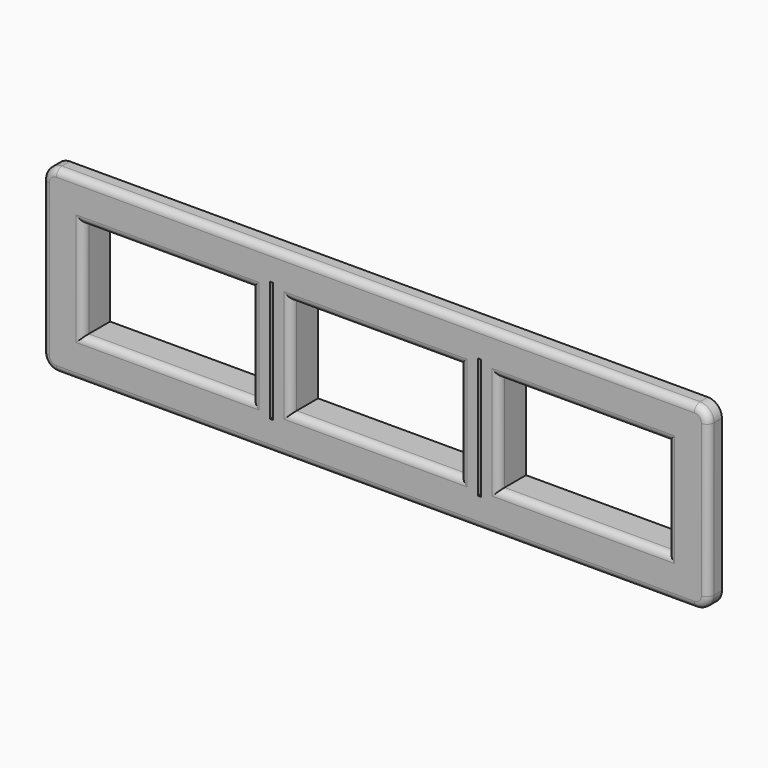
from build123d import *

# Parameters (mm, degrees)
F0_W          = 44.2
F0_H          = 9.6
F0_W_2        = 12
F0_H_2        = 7
F0_W_3        = 0.2
F0_H_3        = 8.6
F1_DEPTH      = 2.4
F2_R          = 0.5
F3_W          = 44.2
F3_H          = 1.2
F4_DEPTH      = 1.6
F5_W          = 44.2
F5_H          = 1.2
F6_DEPTH      = 1.6
F8_DEPTH      = 1.6
F10_DEPTH     = 1.6
F11_R         = 0.5
F12_T1_DEPTH  = 3.7
F12_T3_DEPTH  = 3.7
F12_T6_ANGLE  = 90
F12_T8_ANGLE  = 90
F12_T10_ANGLE = 90
F12_T12_ANGLE = 90


# Not quite as in the source:
# - a fillet or chamfer that OpenCascade refuses, or shapes differently, is made with other operations: its cross-section is extruded or revolved along the edge and cut away or added
# - a feature names something its author has since deleted; it is built from what else it names


with BuildPart() as f1:
    # F0 (on Front) → F1 (new body)
    with BuildSketch(Plane.XZ):
        with Locations((58.0827572465, 2.8)):
            Rectangle(F0_W, F0_H)
        with Locations((43.2827572465, 2.8)):
            Rectangle(F0_W_2, F0_H_2, mode=Mode.SUBTRACT)
        with Locations((50.6827572465, 2.8)):
            Rectangle(F0_W_3, F0_H_3, mode=Mode.SUBTRACT)
        with Locations((58.0827572465, 2.8)):
            Rectangle(F0_W_2, F0_H_2, mode=Mode.SUBTRACT)
        with Locations((65.4827572465, 2.8)):
            Rectangle(F0_W_3, F0_H_3, mode=Mode.SUBTRACT)
        with Locations((72.8827572465, 2.8)):
            Rectangle(F0_W_2, F0_H_2, mode=Mode.SUBTRACT)
    extrude(amount=F1_DEPTH)

    # F2
    f2_edges = [f1.edges().sort_by_distance(p)[0] for p in [
        (43.282757, -2.4, 6.3),
        (37.282757, -2.4, 2.8),
        (49.282757, -2.4, 2.8),
        (58.082757, -2.4, 6.3),
        (52.082757, -2.4, 2.8),
        (58.082757, -2.4, -0.7),
        (43.282757, -2.4, -0.7),
        (64.082757, -2.4, 2.8),
        (66.882757, -2.4, 2.8),
        (72.882757, -2.4, -0.7),
        (72.882757, -2.4, 6.3),
        (78.882757, -2.4, 2.8),
    ]]
    fillet(f2_edges, radius=F2_R)

    # F3 (on face) → F4 (join)
    with BuildSketch(Plane(origin=(0, 0, -2), x_dir=(1, 0, 0), z_dir=(0, 0, -1))):
        with Locations((58.0827572465, 1.8)):
            Rectangle(F3_W, F3_H)
    extrude(amount=F4_DEPTH)

    # F5 (on face) → F6 (join)
    with BuildSketch(Plane.XY.offset(7.6)):
        with Locations((58.0827572465, -1.8)):
            Rectangle(F5_W, F5_H)
    extrude(amount=F6_DEPTH)

    # F7 (on face) → F8 (join)
    with BuildSketch(Plane(origin=(35.9827572465, 0, 0), x_dir=(0, -1, 0), z_dir=(-1, 0, 0))):
        Polygon((2.4, -3.6), (2.4, 9.2), (1.2, 9.2), (1.2, 7.6), (1.2, -2), (1.2, -3.6), align=None)
    extrude(amount=F8_DEPTH)

    # F9 (on face) → F10 (join)
    with BuildSketch(Plane.YZ.offset(80.1827572465)):
        Polygon((-1.2, 9.2), (-2.4, 9.2), (-2.4, -3.6), (-1.2, -3.6), (-1.2, -2), (-1.2, 7.6), align=None)
    extrude(amount=F10_DEPTH)

    # F11
    f11_edges = [f1.edges().sort_by_distance(p)[0] for p in [
        (58.082757, -2.4, 9.2),
        (81.782757, -2.4, 2.8),
        (58.082757, -2.4, -3.6),
        (34.382757, -2.4, 2.8),
    ]]
    fillet(f11_edges, radius=F11_R)

    # F12: fillet of radius 1 on 8 edges, made by hand

    # F12_s2 → F12_t1 (cut)
    with BuildSketch(Plane.XZ.offset(-2.5)):
        with BuildLine():
            ThreePointArc((36.9827572465, 7.6), (36.2756504653, 7.3071067812), (35.9827572465, 6.6))
            Line((35.9827572465, 6.6), (35.9827572465, 7.6))
            Line((35.9827572465, 7.6), (36.9827572465, 7.6))
        make_face()
        with BuildLine():
            ThreePointArc((35.9827572465, -1), (36.2756504653, -1.7071067812), (36.9827572465, -2))
            Line((36.9827572465, -2), (35.9827572465, -2))
            Line((35.9827572465, -2), (35.9827572465, -1))
        make_face()
        with BuildLine():
            ThreePointArc((80.1827572465, -1), (79.8898640277, -1.7071067812), (79.1827572465, -2))
            Line((79.1827572465, -2), (80.1827572465, -2))
            Line((80.1827572465, -2), (80.1827572465, -1))
        make_face()
        with BuildLine():
            ThreePointArc((80.1827572465, 6.6), (79.8898640277, 7.3071067812), (79.1827572465, 7.6))
            Line((79.1827572465, 7.6), (80.1827572465, 7.6))
            Line((80.1827572465, 7.6), (80.1827572465, 6.6))
        make_face()
    extrude(amount=F12_T1_DEPTH, mode=Mode.SUBTRACT)

    # F12_s4 → F12_t3 (cut)
    with BuildSketch(Plane.XZ.offset(-1.3)):
        with BuildLine():
            ThreePointArc((80.7827572465, 9.2), (81.4898640277, 8.9071067812), (81.7827572465, 8.2))
            Line((81.7827572465, 8.2), (81.7827572465, 9.2))
            Line((81.7827572465, 9.2), (80.7827572465, 9.2))
        make_face()
        with BuildLine():
            ThreePointArc((81.7827572465, -2.6), (81.4898640277, -3.3071067812), (80.7827572465, -3.6))
            Line((80.7827572465, -3.6), (81.7827572465, -3.6))
            Line((81.7827572465, -3.6), (81.7827572465, -2.6))
        make_face()
        with BuildLine():
            ThreePointArc((34.3827572465, -2.6), (34.6756504653, -3.3071067812), (35.3827572465, -3.6))
            Line((35.3827572465, -3.6), (34.3827572465, -3.6))
            Line((34.3827572465, -3.6), (34.3827572465, -2.6))
        make_face()
        with BuildLine():
            ThreePointArc((35.3827572465, 9.2), (34.6756504653, 8.9071067812), (34.3827572465, 8.2))
            Line((34.3827572465, 8.2), (34.3827572465, 9.2))
            Line((34.3827572465, 9.2), (35.3827572465, 9.2))
        make_face()
    extrude(amount=F12_T3_DEPTH, mode=Mode.SUBTRACT)

    # F12_s5 → F12_t6 (revolve, cut)
    with BuildSketch(Plane.YZ.offset(35.3827572465)):
        with BuildLine():
            ThreePointArc((-2.4, 8.7), (-2.2535533906, 9.0535533906), (-1.9, 9.2))
            Line((-1.9, 9.2), (-2.4, 9.2))
            Line((-2.4, 9.2), (-2.4, 8.7))
        make_face()
    revolve(axis=Axis((35.3827572465, -2.4, 8.2), (0, -1, 0)), revolution_arc=F12_T6_ANGLE, mode=Mode.SUBTRACT)

    # F12_s7 → F12_t8 (revolve, cut)
    with BuildSketch(Plane.XY.offset(-2.6)):
        with BuildLine():
            ThreePointArc((34.8827572465, -2.4), (34.5292038559, -2.2535533906), (34.3827572465, -1.9))
            Line((34.3827572465, -1.9), (34.3827572465, -2.4))
            Line((34.3827572465, -2.4), (34.8827572465, -2.4))
        make_face()
    revolve(axis=Axis((35.3827572465, -2.4, -2.6), (0, -1, 0)), revolution_arc=F12_T8_ANGLE, mode=Mode.SUBTRACT)

    # F12_s9 → F12_t10 (revolve, cut)
    with BuildSketch(Plane.YZ.offset(80.7827572465)):
        with BuildLine():
            ThreePointArc((-2.4, -3.1), (-2.2535533906, -3.4535533906), (-1.9, -3.6))
            Line((-1.9, -3.6), (-2.4, -3.6))
            Line((-2.4, -3.6), (-2.4, -3.1))
        make_face()
    revolve(axis=Axis((80.7827572465, -2.4, -2.6), (0, -1, 0)), revolution_arc=F12_T10_ANGLE, mode=Mode.SUBTRACT)

    # F12_s11 → F12_t12 (revolve, cut)
    with BuildSketch(Plane.XY.offset(8.2)):
        with BuildLine():
            ThreePointArc((81.2827572465, -2.4), (81.6363106371, -2.2535533906), (81.7827572465, -1.9))
            Line((81.7827572465, -1.9), (81.7827572465, -2.4))
            Line((81.7827572465, -2.4), (81.2827572465, -2.4))
        make_face()
    revolve(axis=Axis((80.7827572465, -2.4, 8.2), (0, -1, 0)), revolution_arc=F12_T12_ANGLE, mode=Mode.SUBTRACT)


solid = f1.part
